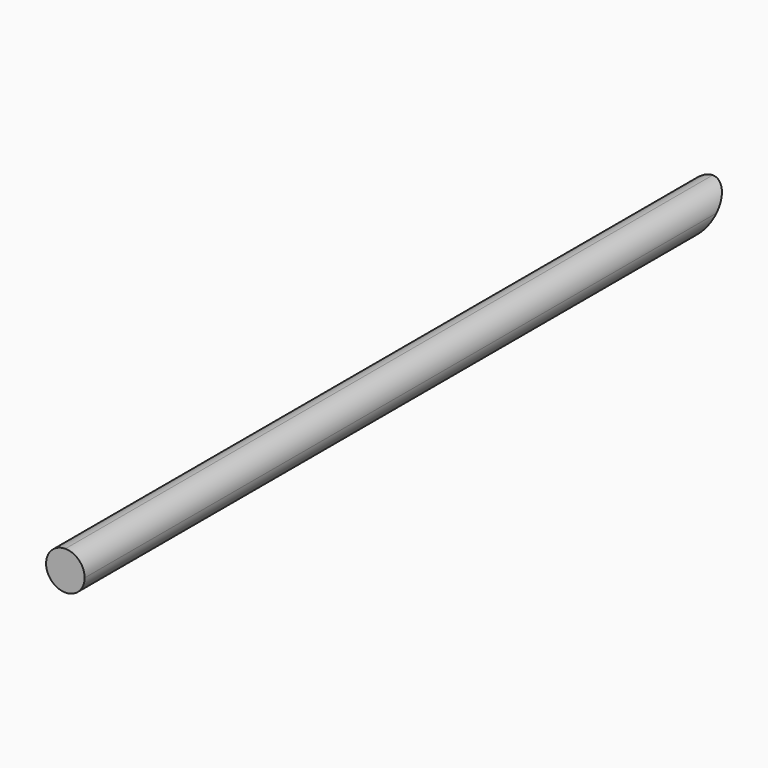
from build123d import *

# Parameters (mm, degrees)
F0_W     = 33
F0_H     = 33
F1_DEPTH = 346
F3_DEPTH = 50
F4_R     = 16.49999


# Not quite as in the source:
# - a fillet or chamfer is up to 0.001 mm smaller than in the source, because OpenCascade refuses the exact size
# - a feature names something its author has since deleted; it is built from what else it names


with BuildPart() as f1:
    # F0 (on Front) → F1 (new body, symmetric)
    with BuildSketch(Plane.XZ):
        Rectangle(F0_W, F0_H)
    extrude(amount=F1_DEPTH, both=True)

    # F2 (on face) → F3 (cut)
    with BuildSketch(Plane.YZ.offset(16.5)):
        Polygon((346, -16.5), (346, 16.5), (313, -16.5), align=None)
    extrude(amount=-F3_DEPTH, mode=Mode.SUBTRACT)

    # F4 (radius 16.5 in the source; OpenCascade refuses exactly that, so slightly less here)
    f4_edges = [f1.edges().sort_by_distance(p)[0] for p in [
        (16.5, 0, 16.5),
        (16.5, -16.5, -16.5),
        (-16.5, -16.5, -16.5),
        (-16.5, 0, 16.5),
    ]]
    fillet(f4_edges, radius=F4_R)


solid = f1.part
